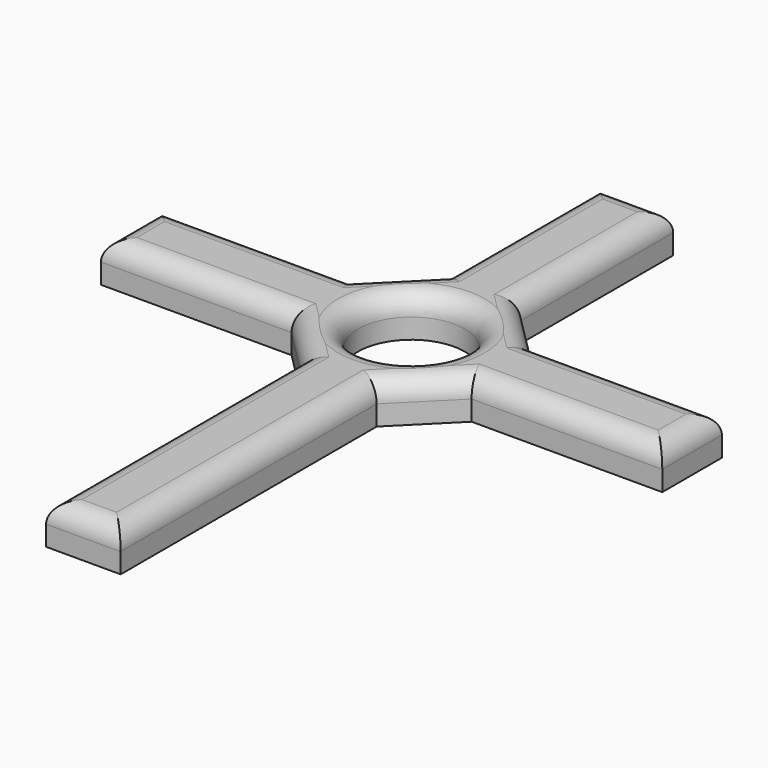
from build123d import *

# Parameters (mm, degrees)
F0_R          = 4
F1_DEPTH      = 3
F2_T1_DEPTH   = 13.091883092
F2_T3_DEPTH   = 13.091883092
F2_T8_DEPTH   = 21.8
F2_T13_DEPTH  = 31.5
F2_T18_DEPTH  = 13.091883092
F2_T24_DEPTH  = 21.8
F2_T29_DEPTH  = 21.8
F2_T34_DEPTH  = 31.5
F2_T39_DEPTH  = 13.091883092
F2_T45_DEPTH  = 13.091883092
F2_T51_DEPTH  = 21.8
F2_T56_DEPTH  = 21.8
F2_T61_DEPTH  = 21.8
F2_T66_DEPTH  = 13.091883092
F2_T75_DEPTH  = 13.091883092
F2_T79_DEPTH  = 21.8
F2_T86_DEPTH  = 31.5
F2_T90_DEPTH  = 13.091883092
F2_T97_DEPTH  = 13.091883092
F2_T101_DEPTH = 21.8
F2_T108_DEPTH = 21.8
F2_T112_DEPTH = 13.091883092
F2_T119_DEPTH = 13.091883092
F2_T123_DEPTH = 31.5
F2_T130_DEPTH = 21.8
F2_T134_DEPTH = 13.091883092
F2_T141_DEPTH = 21.8
F2_T145_DEPTH = 13.091883092
F2_T152_DEPTH = 21.8
F2_T156_DEPTH = 13.091883092


# Not quite as in the source:
# - a fillet or chamfer that OpenCascade refuses, or shapes differently, is made with other operations: its cross-section is extruded or revolved along the edge and cut away or added


with BuildPart() as f1:
    # F0 (on Top) → F1 (new body)
    with BuildSketch(Plane.XY):
        Polygon((-6.75, -2.795941546), (-2.795941546, -6.75), (-2.795941546, -30.75), (2.795941546, -30.75), (2.795941546, -6.75), (6.75, -2.795941546), (21.05, -2.795941546), (21.05, 2.795941546), (6.75, 2.795941546), (2.795941546, 6.75), (2.795941546, 21.05), (-2.795941546, 21.05), (-2.795941546, 6.75), (-6.75, 2.795941546), (-21.05, 2.795941546), (-21.05, -2.795941546), align=None)
        Circle(F0_R, mode=Mode.SUBTRACT)
    extrude(amount=F1_DEPTH)

    # F2: fillet of radius 1.5 on 17 edges, made by hand

    # F2_s2 → F2_t1 (cut)
    with BuildSketch(Plane.XZ.offset(-6.545941546)):
        with BuildLine():
            ThreePointArc((-21.05, 1.5), (-20.6106601718, 2.5606601718), (-19.55, 3))
            Line((-19.55, 3), (-21.05, 3))
            Line((-21.05, 3), (-21.05, 1.5))
        make_face()
        with BuildLine():
            ThreePointArc((21.05, 1.5), (20.6106601718, 2.5606601718), (19.55, 3))
            Line((19.55, 3), (21.05, 3))
            Line((21.05, 3), (21.05, 1.5))
        make_face()
    extrude(amount=F2_T1_DEPTH, mode=Mode.SUBTRACT)

    # F2_s4 → F2_t3 (cut)
    with BuildSketch(Plane.YZ.offset(-6.545941546)):
        with BuildLine():
            ThreePointArc((-30.75, 1.5), (-30.3106601718, 2.5606601718), (-29.25, 3))
            Line((-29.25, 3), (-30.75, 3))
            Line((-30.75, 3), (-30.75, 1.5))
        make_face()
        with BuildLine():
            ThreePointArc((21.05, 1.5), (20.6106601718, 2.5606601718), (19.55, 3))
            Line((19.55, 3), (21.05, 3))
            Line((21.05, 3), (21.05, 1.5))
        make_face()
    extrude(amount=F2_T3_DEPTH, mode=Mode.SUBTRACT)


with BuildPart() as f2_tool6:
    # F2_s7 → F2_t8 (new body)
    with BuildSketch(Plane.YZ.offset(-3)):
        with BuildLine():
            ThreePointArc((2.795941546, 1.5), (2.3566017178, 2.5606601718), (1.295941546, 3))
            Line((1.295941546, 3), (2.795941546, 3))
            Line((2.795941546, 3), (2.795941546, 1.5))
        make_face()
    extrude(amount=-F2_T8_DEPTH)

    split(bisect_by=Plane(origin=(-4.772970773, 4.772970773, 0), x_dir=(0, 0, 1), z_dir=(-0.7071067812, 0.7071067812, 0)), keep=Keep.TOP)


with BuildPart() as f1_1:
    add(f1.part)

    # F2_t5: cut F2_tool6
    add(f2_tool6.part, mode=Mode.SUBTRACT)


with BuildPart() as f2_tool11:
    # F2_s12 → F2_t13 (new body)
    with BuildSketch(Plane.XZ.offset(34.5)):
        with BuildLine():
            ThreePointArc((2.795941546, 1.5), (2.3566017178, 2.5606601718), (1.295941546, 3))
            Line((1.295941546, 3), (2.795941546, 3))
            Line((2.795941546, 3), (2.795941546, 1.5))
        make_face()
    extrude(amount=-F2_T13_DEPTH)

    split(bisect_by=Plane(origin=(4.772970773, -4.772970773, 0), x_dir=(0, 0, 1), z_dir=(0.7071067812, -0.7071067812, 0)), keep=Keep.TOP)


with BuildPart() as f1_2:
    add(f1_1.part)

    # F2_t10: cut F2_tool11
    add(f2_tool11.part, mode=Mode.SUBTRACT)


with BuildPart() as f2_tool16:
    # F2_s17 → F2_t18 (new body)
    with BuildSketch(Plane(origin=(-4.6286796564, -4.6286796564, 0), x_dir=(0, 0, 1), z_dir=(0.7071067812, 0.7071067812, 0))):
        with BuildLine():
            ThreePointArc((1.5, 6.75), (2.5606601718, 6.3106601718), (3, 5.25))
            Line((3, 5.25), (3, 6.75))
            Line((3, 6.75), (1.5, 6.75))
        make_face()
    extrude(amount=F2_T18_DEPTH)

    split(bisect_by=Plane.YZ.offset(2.795941546), keep=Keep.TOP)

    split(bisect_by=Plane.XZ.offset(2.795941546), keep=Keep.TOP)


with BuildPart() as f1_3:
    add(f1_2.part)

    # F2_t15: cut F2_tool16
    add(f2_tool16.part, mode=Mode.SUBTRACT)


with BuildPart() as f2_tool22:
    # F2_s23 → F2_t24 (new body)
    with BuildSketch(Plane.YZ.offset(3)):
        with BuildLine():
            ThreePointArc((-2.795941546, 1.5), (-2.3566017178, 2.5606601718), (-1.295941546, 3))
            Line((-1.295941546, 3), (-2.795941546, 3))
            Line((-2.795941546, 3), (-2.795941546, 1.5))
        make_face()
    extrude(amount=F2_T24_DEPTH)

    split(bisect_by=Plane(origin=(4.772970773, -4.772970773, 0), x_dir=(0, 0, 1), z_dir=(0.7071067812, -0.7071067812, 0)), keep=Keep.TOP)


with BuildPart() as f1_4:
    add(f1_3.part)

    # F2_t21: cut F2_tool22
    add(f2_tool22.part, mode=Mode.SUBTRACT)


with BuildPart() as f2_tool27:
    # F2_s28 → F2_t29 (new body)
    with BuildSketch(Plane.YZ.offset(-24.8)):
        with BuildLine():
            ThreePointArc((-2.795941546, 1.5), (-2.3566017178, 2.5606601718), (-1.295941546, 3))
            Line((-1.295941546, 3), (-2.795941546, 3))
            Line((-2.795941546, 3), (-2.795941546, 1.5))
        make_face()
    extrude(amount=F2_T29_DEPTH)

    split(bisect_by=Plane(origin=(-4.772970773, -4.772970773, 0), x_dir=(0, 0, 1), z_dir=(-0.7071067812, -0.7071067812, 0)), keep=Keep.TOP)


with BuildPart() as f1_5:
    add(f1_4.part)

    # F2_t26: cut F2_tool27
    add(f2_tool27.part, mode=Mode.SUBTRACT)


with BuildPart() as f2_tool32:
    # F2_s33 → F2_t34 (new body)
    with BuildSketch(Plane.XZ.offset(3)):
        with BuildLine():
            ThreePointArc((-2.795941546, 1.5), (-2.3566017178, 2.5606601718), (-1.295941546, 3))
            Line((-1.295941546, 3), (-2.795941546, 3))
            Line((-2.795941546, 3), (-2.795941546, 1.5))
        make_face()
    extrude(amount=F2_T34_DEPTH)

    split(bisect_by=Plane(origin=(-4.772970773, -4.772970773, 0), x_dir=(0, 0, 1), z_dir=(-0.7071067812, -0.7071067812, 0)), keep=Keep.TOP)


with BuildPart() as f1_6:
    add(f1_5.part)

    # F2_t31: cut F2_tool32
    add(f2_tool32.part, mode=Mode.SUBTRACT)


with BuildPart() as f2_tool37:
    # F2_s38 → F2_t39 (new body)
    with BuildSketch(Plane(origin=(-4.6286796564, 4.6286796564, 0), x_dir=(0, 0, 1), z_dir=(0.7071067812, -0.7071067812, 0))):
        with BuildLine():
            ThreePointArc((1.5, 6.75), (2.5606601718, 6.3106601718), (3, 5.25))
            Line((3, 5.25), (3, 6.75))
            Line((3, 6.75), (1.5, 6.75))
        make_face()
    extrude(amount=F2_T39_DEPTH)

    split(bisect_by=Plane.XZ.offset(2.795941546), keep=Keep.TOP)

    split(bisect_by=Plane.YZ.offset(-2.795941546), keep=Keep.BOTTOM)


with BuildPart() as f1_7:
    add(f1_6.part)

    # F2_t36: cut F2_tool37
    add(f2_tool37.part, mode=Mode.SUBTRACT)


with BuildPart() as f2_tool43:
    # F2_s44 → F2_t45 (new body)
    with BuildSketch(Plane(origin=(4.6286796564, 4.6286796564, 0), x_dir=(0, 0, 1), z_dir=(-0.7071067812, -0.7071067812, 0))):
        with BuildLine():
            ThreePointArc((1.5, 6.75), (2.5606601718, 6.3106601718), (3, 5.25))
            Line((3, 5.25), (3, 6.75))
            Line((3, 6.75), (1.5, 6.75))
        make_face()
    extrude(amount=F2_T45_DEPTH)

    split(bisect_by=Plane.YZ.offset(-2.795941546), keep=Keep.BOTTOM)

    split(bisect_by=Plane.XZ.offset(-2.795941546), keep=Keep.BOTTOM)


with BuildPart() as f1_8:
    add(f1_7.part)

    # F2_t42: cut F2_tool43
    add(f2_tool43.part, mode=Mode.SUBTRACT)


with BuildPart() as f2_tool49:
    # F2_s50 → F2_t51 (new body)
    with BuildSketch(Plane.XZ.offset(-24.8)):
        with BuildLine():
            ThreePointArc((-2.795941546, 1.5), (-2.3566017178, 2.5606601718), (-1.295941546, 3))
            Line((-1.295941546, 3), (-2.795941546, 3))
            Line((-2.795941546, 3), (-2.795941546, 1.5))
        make_face()
    extrude(amount=F2_T51_DEPTH)

    split(bisect_by=Plane(origin=(-4.772970773, 4.772970773, 0), x_dir=(0, 0, 1), z_dir=(-0.7071067812, 0.7071067812, 0)), keep=Keep.TOP)


with BuildPart() as f1_9:
    add(f1_8.part)

    # F2_t48: cut F2_tool49
    add(f2_tool49.part, mode=Mode.SUBTRACT)


with BuildPart() as f2_tool54:
    # F2_s55 → F2_t56 (new body)
    with BuildSketch(Plane.XZ.offset(-3)):
        with BuildLine():
            ThreePointArc((2.795941546, 1.5), (2.3566017178, 2.5606601718), (1.295941546, 3))
            Line((1.295941546, 3), (2.795941546, 3))
            Line((2.795941546, 3), (2.795941546, 1.5))
        make_face()
    extrude(amount=-F2_T56_DEPTH)

    split(bisect_by=Plane(origin=(4.772970773, 4.772970773, 0), x_dir=(0, 0, 1), z_dir=(0.7071067812, 0.7071067812, 0)), keep=Keep.TOP)


with BuildPart() as f1_10:
    add(f1_9.part)

    # F2_t53: cut F2_tool54
    add(f2_tool54.part, mode=Mode.SUBTRACT)


with BuildPart() as f2_tool59:
    # F2_s60 → F2_t61 (new body)
    with BuildSketch(Plane.YZ.offset(24.8)):
        with BuildLine():
            ThreePointArc((2.795941546, 1.5), (2.3566017178, 2.5606601718), (1.295941546, 3))
            Line((1.295941546, 3), (2.795941546, 3))
            Line((2.795941546, 3), (2.795941546, 1.5))
        make_face()
    extrude(amount=-F2_T61_DEPTH)

    split(bisect_by=Plane(origin=(4.772970773, 4.772970773, 0), x_dir=(0, 0, 1), z_dir=(0.7071067812, 0.7071067812, 0)), keep=Keep.TOP)


with BuildPart() as f1_11:
    add(f1_10.part)

    # F2_t58: cut F2_tool59
    add(f2_tool59.part, mode=Mode.SUBTRACT)


with BuildPart() as f2_tool64:
    # F2_s65 → F2_t66 (new body)
    with BuildSketch(Plane(origin=(4.6286796564, -4.6286796564, 0), x_dir=(0, 0, 1), z_dir=(-0.7071067812, 0.7071067812, 0))):
        with BuildLine():
            ThreePointArc((1.5, 6.75), (2.5606601718, 6.3106601718), (3, 5.25))
            Line((3, 5.25), (3, 6.75))
            Line((3, 6.75), (1.5, 6.75))
        make_face()
    extrude(amount=F2_T66_DEPTH)

    split(bisect_by=Plane.YZ.offset(2.795941546), keep=Keep.TOP)

    split(bisect_by=Plane.XZ.offset(-2.795941546), keep=Keep.BOTTOM)


with BuildPart() as f1_12:
    add(f1_11.part)

    # F2_t63: cut F2_tool64
    add(f2_tool64.part, mode=Mode.SUBTRACT)

    # F2_s69 → F2_t70 (revolve, cut)
    with BuildSketch(Plane.XZ):
        with BuildLine():
            ThreePointArc((4, 1.5), (4.4393398282, 2.5606601718), (5.5, 3))
            Line((5.5, 3), (4, 3))
            Line((4, 3), (4, 1.5))
        make_face()
    revolve(axis=Axis((0, 0, 3), (0, 0, 1)), mode=Mode.SUBTRACT)


with BuildPart() as f2_tool73:
    # F2_s74 → F2_t75 (new body)
    with BuildSketch(Plane(origin=(4.6286796564, 4.6286796564, 0), x_dir=(0, 0, 1), z_dir=(-0.7071067812, -0.7071067812, 0))):
        with BuildLine():
            ThreePointArc((1.5, 6.75), (2.5606601718, 6.3106601718), (3, 5.25))
            Line((3, 5.25), (3, 6.75))
            Line((3, 6.75), (1.5, 6.75))
        make_face()
    extrude(amount=F2_T75_DEPTH)

    split(bisect_by=Plane.XZ.offset(-2.795941546), keep=Keep.TOP)


with BuildPart() as f2_tool77:
    # F2_s78 → F2_t79 (new body)
    with BuildSketch(Plane.YZ.offset(-3)):
        with BuildLine():
            ThreePointArc((2.795941546, 1.5), (2.3566017178, 2.5606601718), (1.295941546, 3))
            Line((1.295941546, 3), (2.795941546, 3))
            Line((2.795941546, 3), (2.795941546, 1.5))
        make_face()
    extrude(amount=-F2_T79_DEPTH)

    split(bisect_by=Plane(origin=(-4.772970773, 4.772970773, 0), x_dir=(0, 0, 1), z_dir=(0.7071067812, -0.7071067812, 0)), keep=Keep.TOP)


with BuildPart() as f2_tool73_1:
    add(f2_tool73.part)

    # F2_t81: intersect F2_tool77
    add(f2_tool77.part, mode=Mode.INTERSECT)


with BuildPart() as f1_13:
    add(f1_12.part)

    # F2_t71: cut F2_tool73
    add(f2_tool73_1.part, mode=Mode.SUBTRACT)


with BuildPart() as f2_tool84:
    # F2_s85 → F2_t86 (new body)
    with BuildSketch(Plane.XZ.offset(34.5)):
        with BuildLine():
            ThreePointArc((2.795941546, 1.5), (2.3566017178, 2.5606601718), (1.295941546, 3))
            Line((1.295941546, 3), (2.795941546, 3))
            Line((2.795941546, 3), (2.795941546, 1.5))
        make_face()
    extrude(amount=-F2_T86_DEPTH)

    split(bisect_by=Plane(origin=(4.772970773, -4.772970773, 0), x_dir=(0, 0, 1), z_dir=(-0.7071067812, 0.7071067812, 0)), keep=Keep.TOP)


with BuildPart() as f2_tool88:
    # F2_s89 → F2_t90 (new body)
    with BuildSketch(Plane(origin=(-4.6286796564, -4.6286796564, 0), x_dir=(0, 0, 1), z_dir=(0.7071067812, 0.7071067812, 0))):
        with BuildLine():
            ThreePointArc((1.5, 6.75), (2.5606601718, 6.3106601718), (3, 5.25))
            Line((3, 5.25), (3, 6.75))
            Line((3, 6.75), (1.5, 6.75))
        make_face()
    extrude(amount=F2_T90_DEPTH)

    split(bisect_by=Plane.YZ.offset(2.795941546), keep=Keep.BOTTOM)


with BuildPart() as f2_tool84_1:
    add(f2_tool84.part)

    # F2_t92: intersect F2_tool88
    add(f2_tool88.part, mode=Mode.INTERSECT)


with BuildPart() as f1_14:
    add(f1_13.part)

    # F2_t82: cut F2_tool84
    add(f2_tool84_1.part, mode=Mode.SUBTRACT)


with BuildPart() as f2_tool95:
    # F2_s96 → F2_t97 (new body)
    with BuildSketch(Plane(origin=(-4.6286796564, -4.6286796564, 0), x_dir=(0, 0, 1), z_dir=(0.7071067812, 0.7071067812, 0))):
        with BuildLine():
            ThreePointArc((1.5, 6.75), (2.5606601718, 6.3106601718), (3, 5.25))
            Line((3, 5.25), (3, 6.75))
            Line((3, 6.75), (1.5, 6.75))
        make_face()
    extrude(amount=F2_T97_DEPTH)

    split(bisect_by=Plane.XZ.offset(2.795941546), keep=Keep.BOTTOM)


with BuildPart() as f2_tool99:
    # F2_s100 → F2_t101 (new body)
    with BuildSketch(Plane.YZ.offset(3)):
        with BuildLine():
            ThreePointArc((-2.795941546, 1.5), (-2.3566017178, 2.5606601718), (-1.295941546, 3))
            Line((-1.295941546, 3), (-2.795941546, 3))
            Line((-2.795941546, 3), (-2.795941546, 1.5))
        make_face()
    extrude(amount=F2_T101_DEPTH)

    split(bisect_by=Plane(origin=(4.772970773, -4.772970773, 0), x_dir=(0, 0, 1), z_dir=(-0.7071067812, 0.7071067812, 0)), keep=Keep.TOP)


with BuildPart() as f2_tool95_1:
    add(f2_tool95.part)

    # F2_t103: intersect F2_tool99
    add(f2_tool99.part, mode=Mode.INTERSECT)


with BuildPart() as f1_15:
    add(f1_14.part)

    # F2_t93: cut F2_tool95
    add(f2_tool95_1.part, mode=Mode.SUBTRACT)


with BuildPart() as f2_tool106:
    # F2_s107 → F2_t108 (new body)
    with BuildSketch(Plane.YZ.offset(-24.8)):
        with BuildLine():
            ThreePointArc((-2.795941546, 1.5), (-2.3566017178, 2.5606601718), (-1.295941546, 3))
            Line((-1.295941546, 3), (-2.795941546, 3))
            Line((-2.795941546, 3), (-2.795941546, 1.5))
        make_face()
    extrude(amount=F2_T108_DEPTH)

    split(bisect_by=Plane(origin=(-4.772970773, -4.772970773, 0), x_dir=(0, 0, 1), z_dir=(0.7071067812, 0.7071067812, 0)), keep=Keep.TOP)


with BuildPart() as f2_tool110:
    # F2_s111 → F2_t112 (new body)
    with BuildSketch(Plane(origin=(-4.6286796564, 4.6286796564, 0), x_dir=(0, 0, 1), z_dir=(0.7071067812, -0.7071067812, 0))):
        with BuildLine():
            ThreePointArc((1.5, 6.75), (2.5606601718, 6.3106601718), (3, 5.25))
            Line((3, 5.25), (3, 6.75))
            Line((3, 6.75), (1.5, 6.75))
        make_face()
    extrude(amount=F2_T112_DEPTH)

    split(bisect_by=Plane.XZ.offset(2.795941546), keep=Keep.BOTTOM)


with BuildPart() as f2_tool106_1:
    add(f2_tool106.part)

    # F2_t114: intersect F2_tool110
    add(f2_tool110.part, mode=Mode.INTERSECT)


with BuildPart() as f1_16:
    add(f1_15.part)

    # F2_t104: cut F2_tool106
    add(f2_tool106_1.part, mode=Mode.SUBTRACT)


with BuildPart() as f2_tool117:
    # F2_s118 → F2_t119 (new body)
    with BuildSketch(Plane(origin=(-4.6286796564, 4.6286796564, 0), x_dir=(0, 0, 1), z_dir=(0.7071067812, -0.7071067812, 0))):
        with BuildLine():
            ThreePointArc((1.5, 6.75), (2.5606601718, 6.3106601718), (3, 5.25))
            Line((3, 5.25), (3, 6.75))
            Line((3, 6.75), (1.5, 6.75))
        make_face()
    extrude(amount=F2_T119_DEPTH)

    split(bisect_by=Plane.YZ.offset(-2.795941546), keep=Keep.TOP)


with BuildPart() as f2_tool121:
    # F2_s122 → F2_t123 (new body)
    with BuildSketch(Plane.XZ.offset(3)):
        with BuildLine():
            ThreePointArc((-2.795941546, 1.5), (-2.3566017178, 2.5606601718), (-1.295941546, 3))
            Line((-1.295941546, 3), (-2.795941546, 3))
            Line((-2.795941546, 3), (-2.795941546, 1.5))
        make_face()
    extrude(amount=F2_T123_DEPTH)

    split(bisect_by=Plane(origin=(-4.772970773, -4.772970773, 0), x_dir=(0, 0, 1), z_dir=(0.7071067812, 0.7071067812, 0)), keep=Keep.TOP)


with BuildPart() as f2_tool117_1:
    add(f2_tool117.part)

    # F2_t125: intersect F2_tool121
    add(f2_tool121.part, mode=Mode.INTERSECT)


with BuildPart() as f1_17:
    add(f1_16.part)

    # F2_t115: cut F2_tool117
    add(f2_tool117_1.part, mode=Mode.SUBTRACT)


with BuildPart() as f2_tool128:
    # F2_s129 → F2_t130 (new body)
    with BuildSketch(Plane.XZ.offset(-24.8)):
        with BuildLine():
            ThreePointArc((-2.795941546, 1.5), (-2.3566017178, 2.5606601718), (-1.295941546, 3))
            Line((-1.295941546, 3), (-2.795941546, 3))
            Line((-2.795941546, 3), (-2.795941546, 1.5))
        make_face()
    extrude(amount=F2_T130_DEPTH)

    split(bisect_by=Plane(origin=(-4.772970773, 4.772970773, 0), x_dir=(0, 0, 1), z_dir=(0.7071067812, -0.7071067812, 0)), keep=Keep.TOP)


with BuildPart() as f2_tool132:
    # F2_s133 → F2_t134 (new body)
    with BuildSketch(Plane(origin=(4.6286796564, 4.6286796564, 0), x_dir=(0, 0, 1), z_dir=(-0.7071067812, -0.7071067812, 0))):
        with BuildLine():
            ThreePointArc((1.5, 6.75), (2.5606601718, 6.3106601718), (3, 5.25))
            Line((3, 5.25), (3, 6.75))
            Line((3, 6.75), (1.5, 6.75))
        make_face()
    extrude(amount=F2_T134_DEPTH)

    split(bisect_by=Plane.YZ.offset(-2.795941546), keep=Keep.TOP)


with BuildPart() as f2_tool128_1:
    add(f2_tool128.part)

    # F2_t136: intersect F2_tool132
    add(f2_tool132.part, mode=Mode.INTERSECT)


with BuildPart() as f1_18:
    add(f1_17.part)

    # F2_t126: cut F2_tool128
    add(f2_tool128_1.part, mode=Mode.SUBTRACT)


with BuildPart() as f2_tool139:
    # F2_s140 → F2_t141 (new body)
    with BuildSketch(Plane.XZ.offset(-3)):
        with BuildLine():
            ThreePointArc((2.795941546, 1.5), (2.3566017178, 2.5606601718), (1.295941546, 3))
            Line((1.295941546, 3), (2.795941546, 3))
            Line((2.795941546, 3), (2.795941546, 1.5))
        make_face()
    extrude(amount=-F2_T141_DEPTH)

    split(bisect_by=Plane(origin=(4.772970773, 4.772970773, 0), x_dir=(0, 0, 1), z_dir=(-0.7071067812, -0.7071067812, 0)), keep=Keep.TOP)


with BuildPart() as f2_tool143:
    # F2_s144 → F2_t145 (new body)
    with BuildSketch(Plane(origin=(4.6286796564, -4.6286796564, 0), x_dir=(0, 0, 1), z_dir=(-0.7071067812, 0.7071067812, 0))):
        with BuildLine():
            ThreePointArc((1.5, 6.75), (2.5606601718, 6.3106601718), (3, 5.25))
            Line((3, 5.25), (3, 6.75))
            Line((3, 6.75), (1.5, 6.75))
        make_face()
    extrude(amount=F2_T145_DEPTH)

    split(bisect_by=Plane.YZ.offset(2.795941546), keep=Keep.BOTTOM)


with BuildPart() as f2_tool139_1:
    add(f2_tool139.part)

    # F2_t147: intersect F2_tool143
    add(f2_tool143.part, mode=Mode.INTERSECT)


with BuildPart() as f1_19:
    add(f1_18.part)

    # F2_t137: cut F2_tool139
    add(f2_tool139_1.part, mode=Mode.SUBTRACT)


with BuildPart() as f2_tool150:
    # F2_s151 → F2_t152 (new body)
    with BuildSketch(Plane.YZ.offset(24.8)):
        with BuildLine():
            ThreePointArc((2.795941546, 1.5), (2.3566017178, 2.5606601718), (1.295941546, 3))
            Line((1.295941546, 3), (2.795941546, 3))
            Line((2.795941546, 3), (2.795941546, 1.5))
        make_face()
    extrude(amount=-F2_T152_DEPTH)

    split(bisect_by=Plane(origin=(4.772970773, 4.772970773, 0), x_dir=(0, 0, 1), z_dir=(-0.7071067812, -0.7071067812, 0)), keep=Keep.TOP)


with BuildPart() as f2_tool154:
    # F2_s155 → F2_t156 (new body)
    with BuildSketch(Plane(origin=(4.6286796564, -4.6286796564, 0), x_dir=(0, 0, 1), z_dir=(-0.7071067812, 0.7071067812, 0))):
        with BuildLine():
            ThreePointArc((1.5, 6.75), (2.5606601718, 6.3106601718), (3, 5.25))
            Line((3, 5.25), (3, 6.75))
            Line((3, 6.75), (1.5, 6.75))
        make_face()
    extrude(amount=F2_T156_DEPTH)

    split(bisect_by=Plane.XZ.offset(-2.795941546), keep=Keep.TOP)


with BuildPart() as f2_tool150_1:
    add(f2_tool150.part)

    # F2_t158: intersect F2_tool154
    add(f2_tool154.part, mode=Mode.INTERSECT)


with BuildPart() as f1_20:
    add(f1_19.part)

    # F2_t148: cut F2_tool150
    add(f2_tool150_1.part, mode=Mode.SUBTRACT)


solid = f1_20.part
